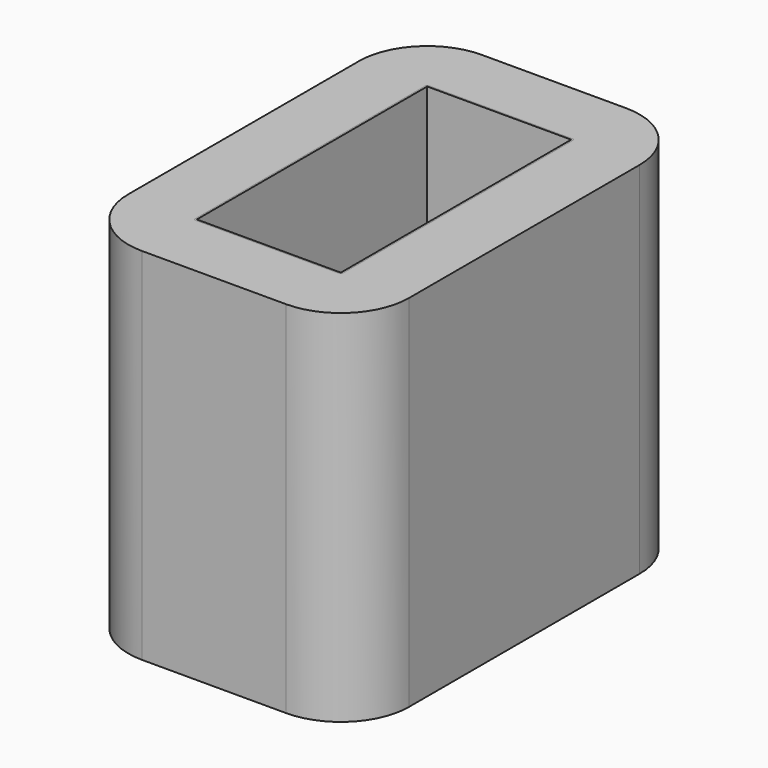
from build123d import *

# Parameters (mm, degrees)
F4_W      = 118.872
F4_H      = 179.832
F5_DEPTH  = 152.4
F6_R      = 28.956
F7_W      = 62.484
F7_H      = 123.444
F8_DEPTH  = 152.4
F9_W      = 62.484
F9_H      = 123.444
F10_DEPTH = 152.4
F11_W     = 60.96
F11_H     = 121.92
F12_DEPTH = 152.4
F13_R     = 0.762
F14_R     = 0.762


# Not quite as in the source:
# - a variable given as a bare number and used for a length is read in inches; the dataset says mm whatever the document's units were


with BuildPart() as f5:
    # F4 (on Top) → F5 (new body)
    with BuildSketch(Plane.XY):
        Rectangle(F4_W, F4_H)
    extrude(amount=-F5_DEPTH)

    # F6
    f6_edges = [f5.edges().sort_by_distance(p)[0] for p in [
        (-59.436, 89.916, -76.2),
        (59.436, 89.916, -76.2),
        (59.436, -89.916, -76.2),
        (-59.436, -89.916, -76.2),
    ]]
    fillet(f6_edges, radius=F6_R)

    # F7 (on face) → F8 (cut)
    with BuildSketch(Plane.XY):
        Rectangle(F7_W, F7_H)
    extrude(amount=-F8_DEPTH, mode=Mode.SUBTRACT)

    # F14
    f14_edges = [f5.edges().sort_by_distance(p)[0] for p in [
        (-31.242, 61.722, -76.2),
        (-31.242, -61.722, -76.2),
        (31.242, -61.722, -76.2),
        (31.242, 61.722, -76.2),
    ]]
    fillet(f14_edges, radius=F14_R)


with BuildPart() as f10:
    # F9 (on face) → F10 (new body)
    with BuildSketch(Plane.XY):
        Rectangle(F9_W, F9_H)
    extrude(amount=-F10_DEPTH)

    # F11 (on face) → F12 (cut)
    with BuildSketch(Plane.XY):
        Rectangle(F11_W, F11_H)
    extrude(amount=-F12_DEPTH, mode=Mode.SUBTRACT)

    # F13
    f13_edges = [f10.edges().sort_by_distance(p)[0] for p in [
        (-31.242, 61.722, -76.2),
        (31.242, 61.722, -76.2),
        (31.242, -61.722, -76.2),
        (-31.242, -61.722, -76.2),
    ]]
    fillet(f13_edges, radius=F13_R)


solid = Compound([f5.part, f10.part])
